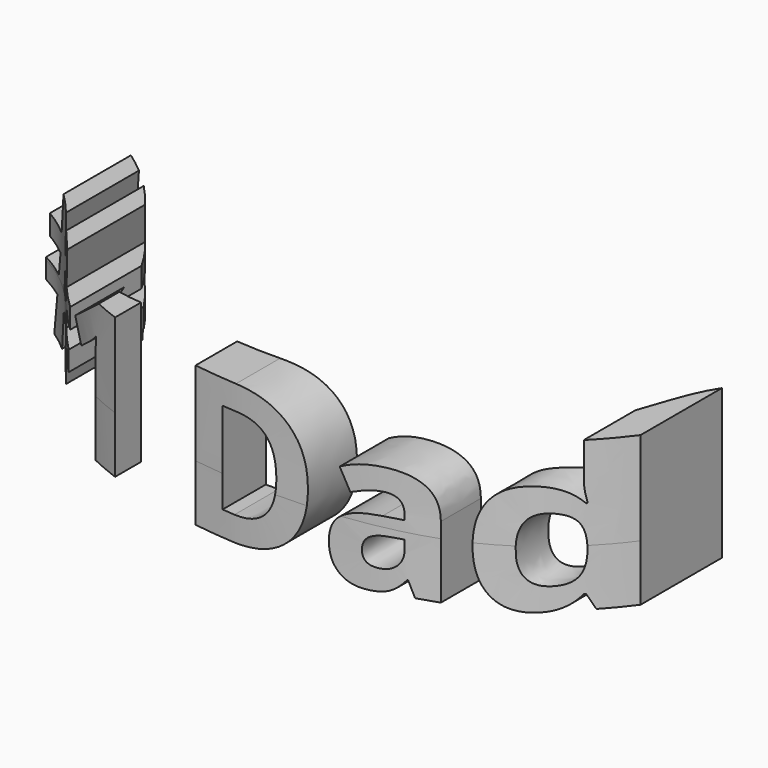
from build123d import *

# Parameters (mm, degrees)
F0_TEXT_SIZE = 9.299791118
F1_DEPTH     = 10
F3_DEPTH     = 12.7
F4_DEPTH     = 12.7


# Not quite as in the source:
# - Text() gives the source's letters only with a copy of the font that has no kerning and outlines rounded to 1/6400 em; it was checked with that copy


with BuildPart() as f1:
    # F0 (on Front) → F1 (new body, symmetric)
    with BuildSketch(Plane.XZ):
        with Locations((-14.8057621602, -2.6640903919)):
            Text('#1 Dad', F0_TEXT_SIZE, font='Open Sans', font_style=FontStyle.BOLD, text_align=(TextAlign.LEFT, TextAlign.BOTTOM))
    extrude(amount=F1_DEPTH, both=True)

    # F2 (on Top) → F3 (cut, symmetric)
    with BuildSketch(Plane.XY):
        with BuildLine():
            add(Edge.make_bspline(
                [(-26.0069089824, 6.6438906289), (-20.6887920245, 5.2834565938), (-12.359459039, 4.0825413224), (-8.8159899827, -5.6247273349), (11.7324239594, -7.4997756845), (18.128072811, 1.264408176), (19.7528415118, 6.2783544051), (29.849322028, 4.316945987), (31.0060671403, 6.5752325035)],
                knots=[0, 0, 0, 0, 0.1894233447, 0.3421022396, 0.562712899, 0.7245763775, 0.8344033827, 1, 1, 1, 1], degree=3))
            Line((-26.0069089824, 6.6438906289), (-27.5842119008, -10.4820011184))
            Line((-27.5842119008, -10.4820011184), (29.3771848083, -10.4820011184))
            Line((29.3771848083, -10.4820011184), (31.0060671403, 6.5752325035))
        make_face()
    extrude(amount=F3_DEPTH, both=True, mode=Mode.SUBTRACT)

    # F2 (on Top) → F4 (cut, symmetric)
    with BuildSketch(Plane.XY):
        with BuildLine():
            Line((26.5163518488, 11.4780580625), (-24.3765875723, 9.7415382772))
            add(Edge.make_bspline(
                [(-24.3765875723, 9.7415382772), (-22.3872776797, 7.306975753), (-15.3629709825, 9.2142335271), (-7.7941474747, 1.8340255862), (-8.2518357439, -3.3394600822), (-2.2074620036, -3.063800055), (1.4990932872, -3.6138852634), (6.8436448273, -2.8631009673), (15.3143920074, -2.6975406338), (15.5715572781, 5.4765638008), (22.2963042249, 7.0588482012), (25.8365499928, 5.5052716975), (27.0801410668, 7.2198956953)],
                knots=[0, 0, 0, 0, 0.122283236, 0.2479887375, 0.3293807602, 0.4194227272, 0.5008393215, 0.5971336006, 0.707251964, 0.8104889538, 0.9095500297, 1, 1, 1, 1], degree=3))
            Line((27.0801410668, 7.2198956953), (26.5163518488, 11.4780580625))
        make_face()
    extrude(amount=F4_DEPTH, both=True, mode=Mode.SUBTRACT)


solid = f1.part
